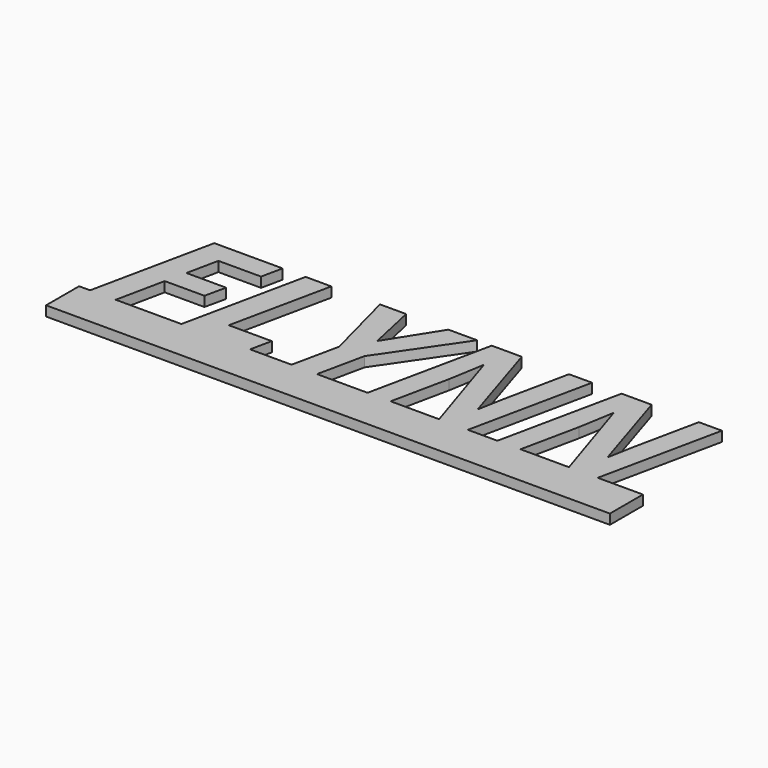
from build123d import *

# Parameters (mm, degrees)
F0_TEXT_SIZE = 34.6502612552
F1_DEPTH     = 2


# Not quite as in the source:
# - Text() gives the source's letters only with a copy of the font that has no kerning and outlines rounded to 1/6400 em; it was checked with that copy


with BuildPart() as f1:
    # F0 (on Top) → F1 (new body)
    with BuildSketch(Plane.XY):
        Polygon((-33.6289219902, 13.8221038505), (-35.8405150473, 13.8221038505), (-35.8405150473, 5.5060405284), (77.7211263776, 5.5060405284), (77.7211263776, 13.8221038505), (68.6110051259, 13.8221038505), (62.8233286756, 13.8221038505), (53.0617003876, 13.8221038505), (48.4109856348, 13.8221038505), (42.4554719816, 13.8221038505), (36.6677955313, 13.8221038505), (26.9061672433, 13.8221038505), (22.2554524905, 13.8221038505), (12.0715241434, 13.8221038505), (6.9443682983, 13.8221038505), (-1.4150072295, 13.8221038505), (-15.2372130083, 13.8221038505), (-28.4692815252, 13.8221038505), align=None)
        with Locations((-34.5276631415, 13.8221038505)):
            Text('FLYNN', F0_TEXT_SIZE, font='Open Sans', font_style=FontStyle.BOLDITALIC, text_align=(TextAlign.LEFT, TextAlign.BOTTOM))
    extrude(amount=F1_DEPTH)


solid = f1.part
